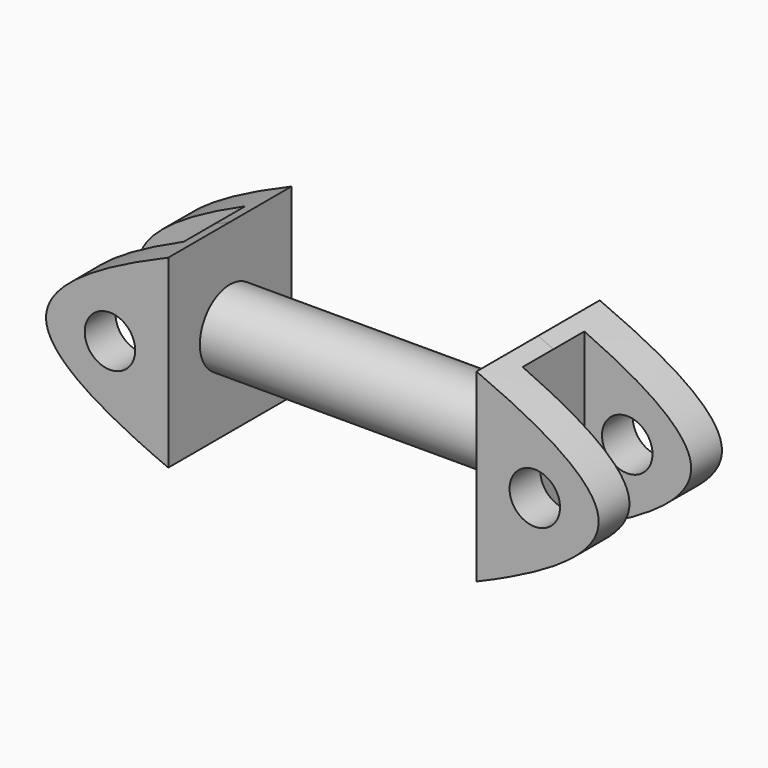
from build123d import *

# Parameters (mm, degrees)
F2_R     = 8.189749857
F3_DEPTH = 25
F5_DEPTH = 12.5


with BuildPart() as f1:
    # F0 (on Front) → F1 (revolve)
    with BuildSketch(Plane.XZ):
        Polygon((0, 12.1819740161), (-50, 12.1819740161), (-50, 0), (50, 0), (50, 12.1819740161), align=None)
    revolve(axis=Axis((74.9588809907, 0, 0), (-1, 0, 0)))

    # F2 (on Front) → F3 (join, symmetric)
    with BuildSketch(Plane.XZ):
        with BuildLine():
            Line((-50, -30), (-50, 30))
            add(Edge.make_bspline(
                [(-50, 30), (-73.5387891531, 20), (-105.7427436113, 0), (-73.5387891531, -20), (-50, -30)],
                knots=[0, 0, 0, 0, 0.5, 1, 1, 1, 1], degree=3))
        make_face()
        with Locations((-68.91708076, 0)):
            Circle(F2_R, mode=Mode.SUBTRACT)
        with BuildLine():
            add(Edge.make_bspline(
                [(50, 30), (73.5387891531, 20), (105.7427436113, 0), (73.5387891531, -20), (50, -30)],
                knots=[0, 0, 0, 0, 0.5, 1, 1, 1, 1], degree=3))
            Line((50, 30), (50, -30))
        make_face()
        with Locations((68.91708076, 0)):
            Circle(F2_R, mode=Mode.SUBTRACT)
    extrude(amount=F3_DEPTH, both=True)

    # F4 (on Front) → F5 (cut, symmetric)
    with BuildSketch(Plane.XZ):
        with BuildLine():
            Line((-55, -27.8246053089), (-55, 27.8246053089))
            add(Edge.make_bspline(
                [(-55, 27.8246053089), (-75.7893328005, 18.5497368726), (-103.492199964, -1e-10), (-75.7893328003, -18.5497368728), (-54.9999999995, -27.8246053091)],
                knots=[0.0362565782, 0.0362565782, 0.0362565782, 0.0362565782, 0.5, 0.9637434218, 0.9637434218, 0.9637434218, 0.9637434218], degree=3))
        make_face()
        with BuildLine():
            add(Edge.make_bspline(
                [(55, 27.8246053089), (75.7893328005, 18.5497368726), (103.492199964, -1e-10), (75.7893328003, -18.5497368728), (54.9999999995, -27.8246053091)],
                knots=[0.0362565782, 0.0362565782, 0.0362565782, 0.0362565782, 0.5, 0.9637434218, 0.9637434218, 0.9637434218, 0.9637434218], degree=3))
            Line((55, 27.8246053089), (55, -27.8246053089))
        make_face()
    extrude(amount=F5_DEPTH, both=True, mode=Mode.SUBTRACT)


solid = f1.part
